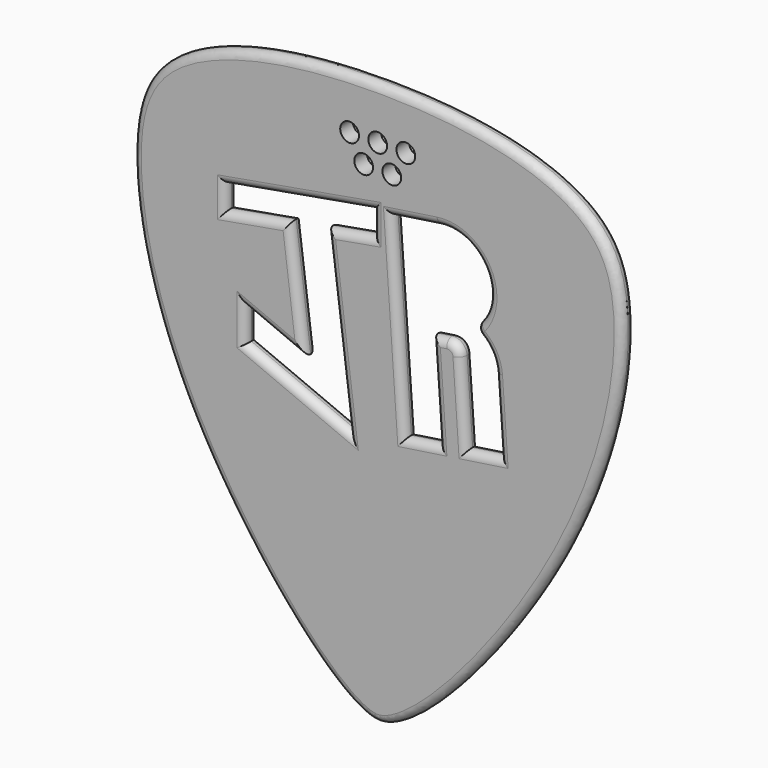
from build123d import *

# Parameters (mm, degrees)
F0_R     = 0.5
F1_DEPTH = 0.84
F2_R     = 0.4199
F3_R     = 0.41999


# Not quite as in the source:
# - a fillet or chamfer is up to 0.001 mm smaller than in the source, because OpenCascade refuses the exact size


with BuildPart() as f1:
    # F0 (on Front) → F1 (new body)
    with BuildSketch(Plane.XZ):
        with BuildLine():
            add(Edge.make_bspline(
                [(0, -23.25), (-2, -23.25), (-11.2052838081, -12.6454945316), (-13.7939030188, -0.3656097413), (-11.4819416014, 5.2828342286), (-5, 6.75), (0, 6.75)],
                knots=[0, 0, 0, 0, 0.2911366771, 0.5724636983, 0.7401439848, 1, 1, 1, 1], degree=3))
            add(Edge.make_bspline(
                [(0, -23.25), (2, -23.25), (11.2052838081, -12.6454945316), (13.7939030188, -0.3656097413), (11.4819416014, 5.2828342286), (5, 6.75), (0, 6.75)],
                knots=[0, 0, 0, 0, 0.2911366771, 0.5724636983, 0.7401439848, 1, 1, 1, 1], degree=3))
        make_face()
        Polygon((-0.25, -0.5), (-2.7097485316, -0.9337200319), (-1.542408067, -10.1097658164), (-7.0756138971, -7.7895000466), (-7.0756138971, -6.0395000466), (-3.9073137099, -7.3680785775), (-4.6816348886, -1.2814167995), (-8.1284620241, -1.8891854213), (-8.1284620241, -0.6391854213), (-0.25, 0.75), align=None, mode=Mode.SUBTRACT)
        with Locations((-0.75, 2.75)):
            Circle(F0_R, mode=Mode.SUBTRACT)
        with Locations((-1.5, 4)):
            Circle(F0_R, mode=Mode.SUBTRACT)
        with BuildLine():
            Line((1.4615160322, -9.4251533127), (0.75, 0.75))
            Line((0.75, 0.75), (3.2225739629, 1.1192939179))
            ThreePointArc((3.2225739629, 1.1192939179), (5.7434258747, -0.2851893969), (5.0276366561, -3.0807060821))
            ThreePointArc((5.0276366561, -3.0807060821), (5.868954756, -3.7604366774), (6.2333425349, -4.7788036907))
            Line((6.2333425349, -4.7788036907), (6.5055669166, -8.6717937201))
            Line((6.5055669166, -8.6717937201), (4.7253136633, -8.937685341))
            Line((4.7253136633, -8.937685341), (4.429349864, -4.7052058231))
            ThreePointArc((4.429349864, -4.7052058231), (4.1692268068, -4.2081365611), (3.6276527318, -4.0617146451))
            Line((3.6276527318, -4.0617146451), (2.8929869168, -4.1714414405))
            Line((2.8929869168, -4.1714414405), (3.2417692855, -9.1592616918))
            Line((3.2417692855, -9.1592616918), (1.4615160322, -9.4251533127))
        make_face(mode=Mode.SUBTRACT)
        with BuildLine():
            ThreePointArc((1.25, 2.75), (0.75, 2.25), (0.25, 2.75))
            ThreePointArc((0.25, 2.75), (0.75, 3.25), (1.25, 2.75))
        make_face(mode=Mode.SUBTRACT)
        with BuildLine():
            ThreePointArc((-0.5, 4), (0, 4.5), (0.5, 4))
            ThreePointArc((0.5, 4), (0, 3.5), (-0.5, 4))
        make_face(mode=Mode.SUBTRACT)
        with BuildLine():
            ThreePointArc((2, 4), (1.5, 3.5), (1, 4))
            ThreePointArc((1, 4), (1.5, 4.5), (2, 4))
        make_face(mode=Mode.SUBTRACT)
    extrude(amount=F1_DEPTH)

    # F2 (radius 0.42 in the source; OpenCascade refuses exactly that, so slightly less here)
    f2_edges = [f1.edges().sort_by_distance(p)[0] for p in [
        (-12.350697, -0.84, -5.69865),
        (12.350697, -0.84, -5.69865),
        (-12.350697, 0, -5.69865),
        (12.350697, 0, -5.69865),
    ]]
    fillet(f2_edges, radius=F2_R)

    # F3 (radius 0.42 in the source; OpenCascade refuses exactly that, so slightly less here)
    f3_edges = [f1.edges().sort_by_distance(p)[0] for p in [
        (-5.491464, -0.84, -6.703789),
        (-4.294474, -0.84, -4.324748),
        (-7.075614, -0.84, -6.9145),
        (-4.309011, -0.84, -8.949633),
        (-2.126078, -0.84, -5.521743),
        (-1.479874, -0.84, -0.71686),
        (-0.25, -0.84, 0.125),
        (-4.189231, -0.84, 0.055407),
        (-8.128462, -0.84, -1.264185),
        (-6.405048, -0.84, -1.585301),
        (1.986287, -0.84, 0.934647),
        (5.743426, -0.84, -0.285189),
        (1.105758, -0.84, -4.337577),
        (2.351643, -0.84, -9.292208),
        (3.067378, -0.84, -6.665352),
        (3.26032, -0.84, -4.116578),
        (5.61544, -0.84, -8.80474),
        (6.369455, -0.84, -6.725299),
        (5.868955, -0.84, -3.760437),
        (5.61544, 0, -8.80474),
        (4.577332, 0, -6.821446),
        (6.369455, 0, -6.725299),
        (5.743426, 0, -0.285189),
        (1.986287, 0, 0.934647),
        (1.105758, 0, -4.337577),
        (3.26032, 0, -4.116578),
        (3.067378, 0, -6.665352),
        (2.351643, 0, -9.292208),
        (-2.126078, 0, -5.521743),
        (-4.309011, 0, -8.949633),
        (-7.075614, 0, -6.9145),
        (-5.491464, 0, -6.703789),
        (-4.294474, 0, -4.324748),
        (-6.405048, 0, -1.585301),
        (-8.128462, 0, -1.264185),
        (-4.189231, 0, 0.055407),
        (-1.479874, 0, -0.71686),
        (-0.25, 0, 0.125),
        (5.027637, -0.42, -3.080706),
    ]]
    fillet(f3_edges, radius=F3_R)


solid = f1.part
